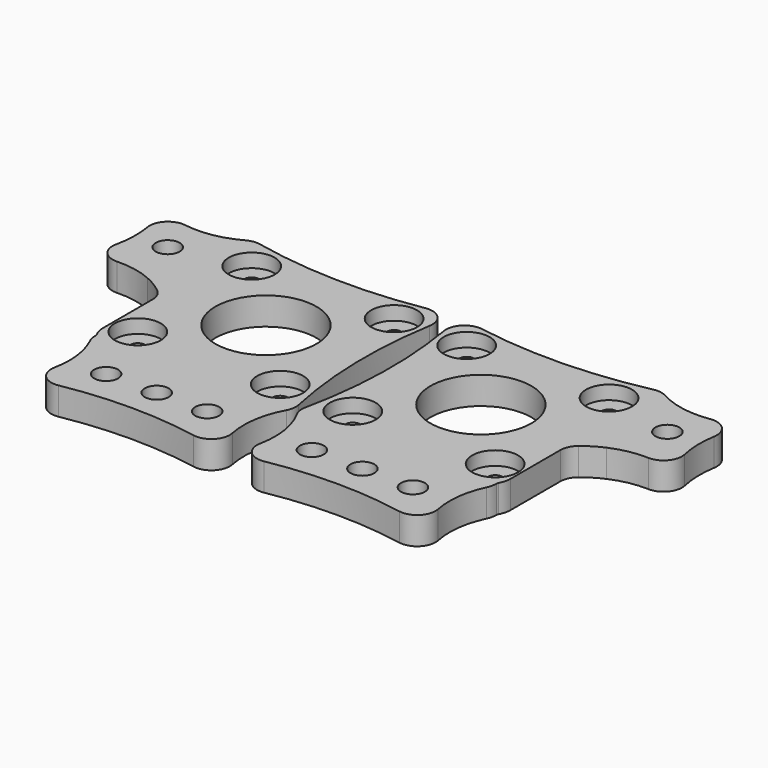
from build123d import *

# Parameters (mm, degrees)
F0_R     = 2.6
F0_R_2   = 5
F0_R_3   = 11
F1_DEPTH = 6
F2_R     = 4
F3_R     = 5
F0_R_4   = 1.6
F4_DEPTH = 3


# Not quite as in the source:
# - a feature names something its author has since deleted; it is built from what else it names


with BuildPart() as f1:
    # F0 (on Top) → F1 (new body)
    with BuildSketch(Plane.XY):
        with BuildLine():
            Line((35.75, -5.5), (-7.5, -5.5))
            ThreePointArc((-7.5, -5.5), (-4.5, -15.5), (-7.5, -25.5))
            ThreePointArc((-7.5, -25.5), (14.5, -22.5), (36.5, -25.5))
            ThreePointArc((36.5, -25.5), (33.5038708252, -15.875), (36.1001689776, -6.134535384))
            ThreePointArc((36.1001689776, -6.134535384), (35.8433519714, -5.8623718623), (35.75, -5.5))
        make_face()
        with Locations((3.5, -15.5)):
            Circle(F0_R, mode=Mode.SUBTRACT)
        with Locations((14.5, -15.5)):
            Circle(F0_R, mode=Mode.SUBTRACT)
        with Locations((25.5, -15.5)):
            Circle(F0_R, mode=Mode.SUBTRACT)
        with BuildLine():
            ThreePointArc((36.5, 38.5), (14.5, 36), (-7.5, 38.5))
            ThreePointArc((-7.5, 38.5), (-5, 16.5), (-7.5, -5.5))
            Line((-7.5, -5.5), (35.75, -5.5))
            ThreePointArc((35.75, -5.5), (35.9696699141, -4.9696699141), (36.5, -4.75))
            Line((36.5, -4.75), (36.5, 12.6569457352))
            Line((36.5, 12.6569457352), (36.5, 16.5))
            Line((36.5, 16.5), (36.5, 38.5))
        make_face()
        Circle(F0_R_2, mode=Mode.SUBTRACT)
        with Locations((31, 0)):
            Circle(F0_R_2, mode=Mode.SUBTRACT)
        with Locations((15.5, 15.5)):
            Circle(F0_R_3, mode=Mode.SUBTRACT)
        with Locations((0, 31)):
            Circle(F0_R_2, mode=Mode.SUBTRACT)
        with Locations((31, 31)):
            Circle(F0_R_2, mode=Mode.SUBTRACT)
        with BuildLine():
            ThreePointArc((56.5, 38.5), (46.5, 35.5), (36.5, 38.5))
            Line((36.5, 38.5), (36.5, 16.5))
            Line((36.5, 16.5), (42.097686123, 16.5))
            ThreePointArc((42.097686123, 16.5), (49.2988430615, 18.0040277618), (56.5, 16.5))
            ThreePointArc((56.5, 16.5), (53.5, 27.5), (56.5, 38.5))
        make_face()
        with Locations((46.5, 27.5)):
            Circle(F0_R, mode=Mode.SUBTRACT)
        with BuildLine():
            Line((42.097686123, 16.5), (36.5, 16.5))
            Line((36.5, 16.5), (36.5, 12.6569457352))
            ThreePointArc((36.5, 12.6569457352), (39.1159030872, 14.8449381541), (42.097686123, 16.5))
        make_face()
    extrude(amount=F1_DEPTH)

    # F2
    f2_edges = [f1.edges().sort_by_distance(p)[0] for p in [
        (36.5, -25.5, 3),
        (-7.5, -25.5, 3),
        (-7.5, 38.5, 3),
        (36.5, 38.5, 3),
        (-7.5, -5.5, 3),
        (56.5, 16.5, 3),
        (36.5, 12.656946, 3),
        (56.5, 38.5, 3),
    ]]
    fillet(f2_edges, radius=F2_R)

    # F3
    f3_edges = [f1.edges().sort_by_distance(p)[0] for p in [
        (36.100169, -6.134535, 3),
        (36.5, -4.75, 3),
    ]]
    fillet(f3_edges, radius=F3_R)

    # F0 (on Top) → F4 (join)
    with BuildSketch(Plane.XY):
        with Locations((0, 31)):
            Circle(F0_R_2)
        with Locations((0, 31)):
            Circle(F0_R_4, mode=Mode.SUBTRACT)
        with Locations((31, 31)):
            Circle(F0_R_2)
        with Locations((31, 31)):
            Circle(F0_R_4, mode=Mode.SUBTRACT)
        Circle(F0_R_2)
        Circle(F0_R_4, mode=Mode.SUBTRACT)
        with Locations((31, 0)):
            Circle(F0_R_2)
        with Locations((31, 0)):
            Circle(F0_R_4, mode=Mode.SUBTRACT)
    extrude(amount=F4_DEPTH)


with BuildPart() as f5_1:
    # F5: instance of F1
    add(f1.part.mirror(Plane.YZ))


with BuildPart() as f5_1_1:
    # F6: moved
    add(f5_1.part.moved(Location((-15.8, 0, 0))))


solid = Compound([f1.part, f5_1_1.part])
